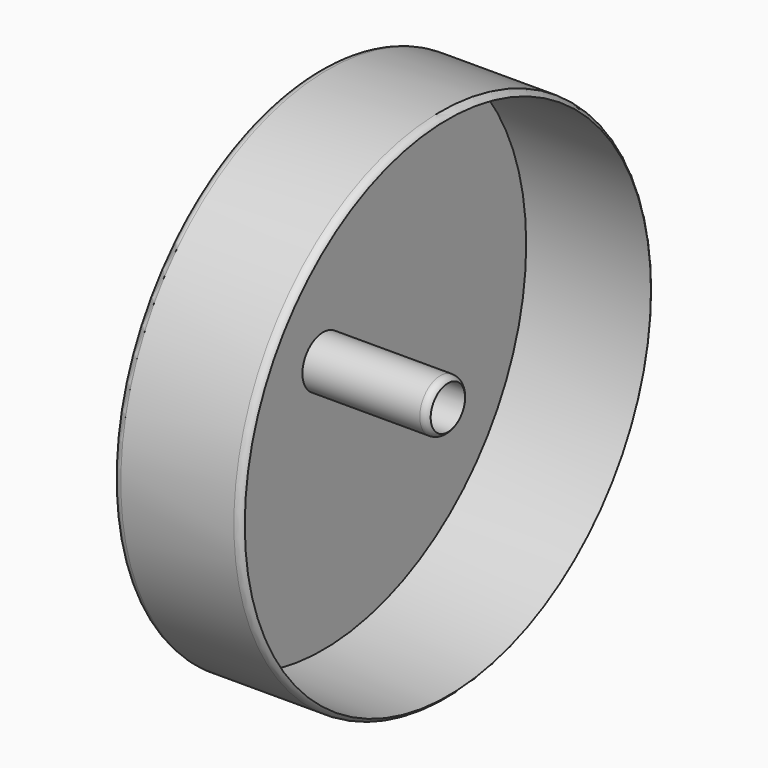
from build123d import *

# Parameters (mm, degrees)
F0_R     = 152.4
F0_R_2   = 12.7
F1_DEPTH = 76.2
F2_T     = -2.54
F4_R     = 5.08


# Not quite as in the source:
# - a fillet or chamfer that OpenCascade refuses, or shapes differently, is made with other operations: its cross-section is extruded or revolved along the edge and cut away or added


with BuildPart() as f1:
    # F0 (on Right) → F1 (new body)
    with BuildSketch(Plane.YZ):
        Circle(F0_R)
        Circle(F0_R_2, mode=Mode.SUBTRACT)
    extrude(amount=F1_DEPTH)

    # F2
    f2_openings = [f1.faces().sort_by_distance(p)[0] for p in [
        (76.2, -148.089477, 0),
    ]]
    offset(amount=F2_T, openings=f2_openings)

    # F3: fillet of radius 5.08 on 2 edges, made by hand

    # F3_s1 → F3_t2 (revolve, cut)
    with BuildSketch(Plane.XY):
        with BuildLine():
            ThreePointArc((71.8005909488, 152.4), (74.3405909488, 151.7194090512), (76.2, 149.86))
            Line((76.2, 149.86), (76.2, 152.4))
            Line((76.2, 152.4), (71.8005909488, 152.4))
        make_face()
    revolve(axis=Axis((76.2, 0, 0), (1, 0, 0)), mode=Mode.SUBTRACT)

    # F3_s3 → F3_t4 (revolve, cut)
    with BuildSketch(Plane.XY):
        with BuildLine():
            ThreePointArc((76.2, 12.7), (74.3405909488, 14.5594090512), (71.8005909488, 15.24))
            Line((71.8005909488, 15.24), (76.2, 15.24))
            Line((76.2, 15.24), (76.2, 12.7))
        make_face()
    revolve(axis=Axis((76.2, 0, 0), (1, 0, 0)), mode=Mode.SUBTRACT)

    # F4
    f4_edges = [f1.edges().sort_by_distance(p)[0] for p in [
        (0, -152.4, 0),
        (35.900295, 152.4, 0),
        (71.800591, -152.4, 0),
    ]]
    fillet(f4_edges, radius=F4_R)


solid = f1.part
